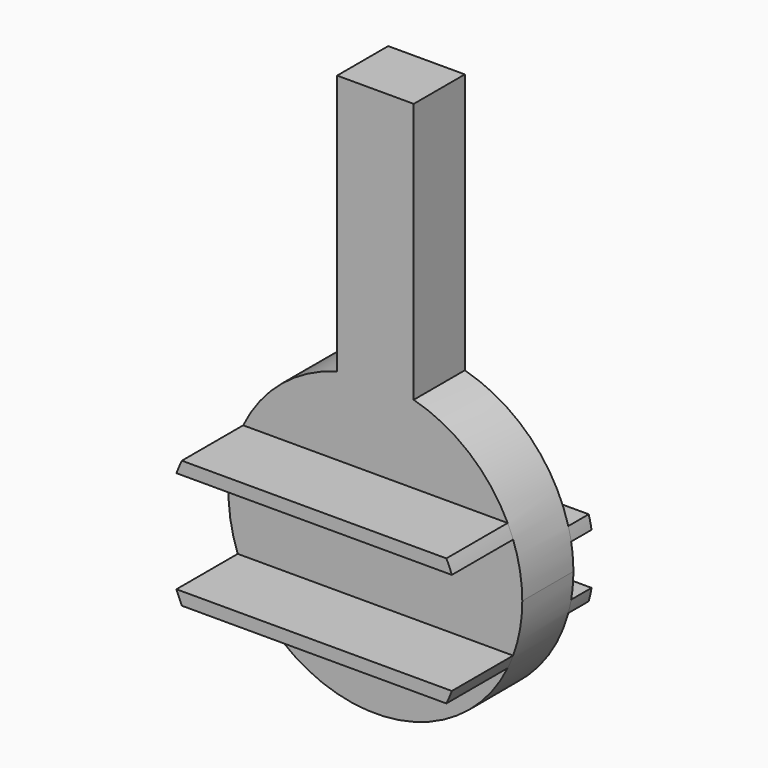
from build123d import *

# Parameters (mm, degrees)
F1_DEPTH = 2.5
F2_W     = 10.3561575886
F2_H     = 0.5
F3_DEPTH = 3
F4_W     = 11.1018016556
F4_H     = 0.5
F5_DEPTH = 1
F6_DEPTH = 2.5
F7_W     = 3
F7_H     = 2.5
F8_DEPTH = 10


# Not quite as in the source:
# - after a boolean that leaves OpenCascade's solid faulty, fix() repairs it


with BuildPart() as f1:
    # F0 (on Front) → F1 (new body)
    with BuildSketch(Plane.XZ):
        with BuildLine():
            ThreePointArc((-1.5, 5.5509008278), (-3.4955328635, -4.5654955919), (5.75, 0))
            ThreePointArc((5.75, 0), (4.5654955919, 3.4955328635), (1.5, 5.5509008278))
            ThreePointArc((1.5, 5.5509008278), (0.7565779009, 5.7000078842), (0, 5.75))
            ThreePointArc((0, 5.75), (-0.7565779009, 5.7000078842), (-1.5, 5.5509008278))
        make_face()
    extrude(amount=F1_DEPTH)

    # F2 (on face) → F3 (join)
    with BuildSketch(Plane.XZ.offset(2.5)):
        with Locations((0, 2.25)):
            Rectangle(F2_W, F2_H)
        with Locations((0, -2.25)):
            Rectangle(F2_W, F2_H)
        with BuildLine():
            Line((5.1780787943, 2.5), (5.1780787943, 2))
            Line((5.1780787943, 2), (5.3909646632, 2))
            ThreePointArc((5.3909646632, 2), (5.2904319201, 2.2525163925), (5.1780787943, 2.5))
        make_face()
        with BuildLine():
            ThreePointArc((-5.1780787943, 2.5), (-5.2904319201, 2.2525163925), (-5.3909646632, 2))
            Line((-5.3909646632, 2), (-5.1780787943, 2))
            Line((-5.1780787943, 2), (-5.1780787943, 2.5))
        make_face()
        with BuildLine():
            Line((-5.1780787943, -2), (-5.3909646632, -2))
            ThreePointArc((-5.3909646632, -2), (-5.2904319201, -2.2525163925), (-5.1780787943, -2.5))
            Line((-5.1780787943, -2.5), (-5.1780787943, -2))
        make_face()
        with BuildLine():
            Line((5.3909646632, -2), (5.1780787943, -2))
            Line((5.1780787943, -2), (5.1780787943, -2.5))
            ThreePointArc((5.1780787943, -2.5), (5.2904319201, -2.2525163925), (5.3909646632, -2))
        make_face()
    extrude(amount=F3_DEPTH)

    # F4 (on face) → F5 (join)
    with BuildSketch(Plane(origin=(0, 0, 0), x_dir=(-1, 0, 0), z_dir=(0, 1, 0))):
        with Locations((0, 1.25)):
            Rectangle(F4_W, F4_H)
        with Locations((0, -1.25)):
            Rectangle(F4_W, F4_H)
        with BuildLine():
            Line((5.5509008278, 1.5), (5.5509008278, 1))
            Line((5.5509008278, 1), (5.6623758265, 1))
            ThreePointArc((5.6623758265, 1), (5.6122093093, 1.2512420505), (5.5509008278, 1.5))
        make_face()
        with BuildLine():
            Line((5.6623758265, -1), (5.5509008278, -1))
            Line((5.5509008278, -1), (5.5509008278, -1.5))
            ThreePointArc((5.5509008278, -1.5), (5.6122093093, -1.2512420505), (5.6623758265, -1))
        make_face()
        with BuildLine():
            Line((-5.5509008278, -1), (-5.6623758265, -1))
            ThreePointArc((-5.6623758265, -1), (-5.6122093093, -1.2512420505), (-5.5509008278, -1.5))
            Line((-5.5509008278, -1.5), (-5.5509008278, -1))
        make_face()
        with BuildLine():
            ThreePointArc((-5.5509008278, 1.5), (-5.6122093093, 1.2512420505), (-5.6623758265, 1))
            Line((-5.6623758265, 1), (-5.5509008278, 1))
            Line((-5.5509008278, 1), (-5.5509008278, 1.5))
        make_face()
    extrude(amount=F5_DEPTH)

    add(f1.part.fix(), mode=Mode.REPLACE)

    # F0 (on Front) → F6 (join)
    with BuildSketch(Plane.XZ):
        with BuildLine():
            ThreePointArc((0, 5.75), (0.7565779009, 5.7000078842), (1.5, 5.5509008278))
            Line((1.5, 5.5509008278), (1.5, 5.75))
            Line((1.5, 5.75), (0, 5.75))
        make_face()
        with BuildLine():
            Line((-1.5, 5.75), (-1.5, 5.5509008278))
            ThreePointArc((-1.5, 5.5509008278), (-0.7565779009, 5.7000078842), (0, 5.75))
            Line((0, 5.75), (-1.5, 5.75))
        make_face()
    extrude(amount=F6_DEPTH)

    # F7 (on face) → F8 (join)
    with BuildSketch(Plane.XY.offset(5.75)):
        with Locations((0, -1.25)):
            Rectangle(F7_W, F7_H)
    extrude(amount=F8_DEPTH)


solid = f1.part
